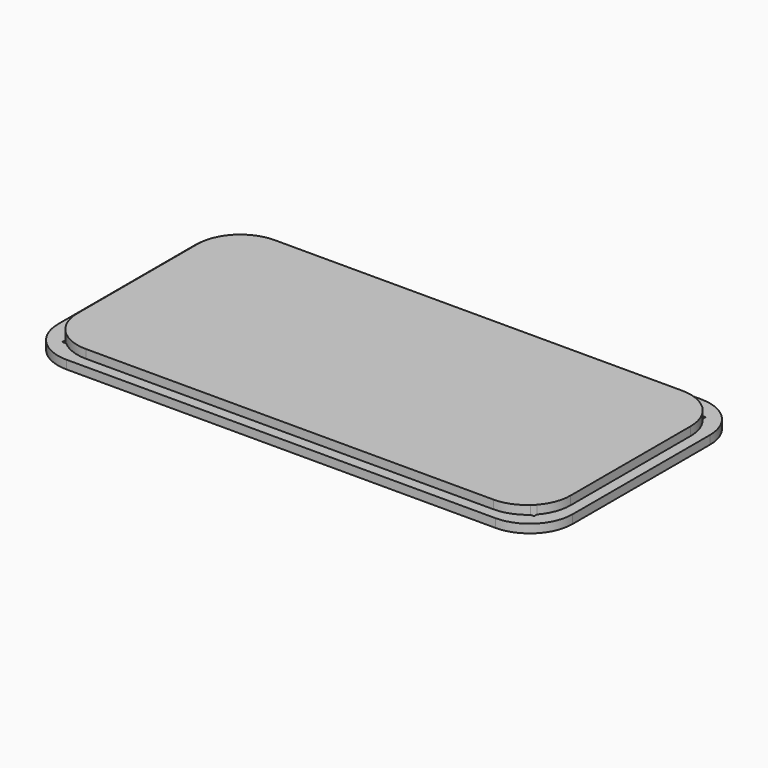
from build123d import *

# Parameters (mm, degrees)
F1_DEPTH = 1
F2_DEPTH = 2


with BuildPart() as f1:
    # F0 (on Top) → F1 (new body)
    with BuildSketch(Plane.XY):
        with BuildLine():
            Line((25, 15), (-25, 15))
            ThreePointArc((-25, 15), (-28.5355339059, 13.5355339059), (-30, 10))
            Line((-30, 10), (-30, -10))
            ThreePointArc((-30, -10), (-28.5355339059, -13.5355339059), (-25, -15))
            Line((-25, -15), (25, -15))
            ThreePointArc((25, -15), (28.5355339059, -13.5355339059), (30, -10))
            Line((30, -10), (30, 10))
            ThreePointArc((30, 10), (28.5355339059, 13.5355339059), (25, 15))
        make_face()
        with BuildLine():
            Line((-27.5, 12.0571891388), (-27.5, 12.5))
            Line((-27.5, 12.5), (-27.0571891388, 12.5))
            ThreePointArc((-27.0571891388, 12.5), (-25.517766953, 13.4270717335), (-23.75, 13.75))
            Line((-23.75, 13.75), (23.75, 13.75))
            ThreePointArc((23.75, 13.75), (25.517766953, 13.4270717335), (27.0571891388, 12.5))
            Line((27.0571891388, 12.5), (27.5, 12.5))
            Line((27.5, 12.5), (27.5, 12.0571891388))
            ThreePointArc((27.5, 12.0571891388), (28.4270717335, 10.517766953), (28.75, 8.75))
            Line((28.75, 8.75), (28.75, -8.75))
            ThreePointArc((28.75, -8.75), (28.4270717335, -10.517766953), (27.5, -12.0571891388))
            Line((27.5, -12.0571891388), (27.5, -12.5))
            Line((27.5, -12.5), (27.0571891388, -12.5))
            ThreePointArc((27.0571891388, -12.5), (25.517766953, -13.4270717335), (23.75, -13.75))
            Line((23.75, -13.75), (-23.75, -13.75))
            ThreePointArc((-23.75, -13.75), (-25.517766953, -13.4270717335), (-27.0571891388, -12.5))
            Line((-27.0571891388, -12.5), (-27.5, -12.5))
            Line((-27.5, -12.5), (-27.5, -12.0571891388))
            ThreePointArc((-27.5, -12.0571891388), (-28.4270717335, -10.517766953), (-28.75, -8.75))
            Line((-28.75, -8.75), (-28.75, 8.75))
            ThreePointArc((-28.75, 8.75), (-28.4270717335, 10.517766953), (-27.5, 12.0571891388))
        make_face(mode=Mode.SUBTRACT)
    extrude(amount=F1_DEPTH)

    # F0 (on Top) → F2 (join)
    with BuildSketch(Plane.XY):
        with BuildLine():
            Line((27.0571891388, 12.5), (-27.0571891388, 12.5))
            ThreePointArc((-27.0571891388, 12.5), (-27.2855339059, 12.2855339059), (-27.5, 12.0571891388))
            Line((-27.5, 12.0571891388), (-27.5, -12.0571891388))
            ThreePointArc((-27.5, -12.0571891388), (-27.2855339059, -12.2855339059), (-27.0571891388, -12.5))
            Line((-27.0571891388, -12.5), (27.0571891388, -12.5))
            ThreePointArc((27.0571891388, -12.5), (27.2855339059, -12.2855339059), (27.5, -12.0571891388))
            Line((27.5, -12.0571891388), (27.5, 12.0571891388))
            ThreePointArc((27.5, 12.0571891388), (27.2855339059, 12.2855339059), (27.0571891388, 12.5))
        make_face()
        with BuildLine():
            ThreePointArc((28.75, 8.75), (28.4270717335, 10.517766953), (27.5, 12.0571891388))
            Line((27.5, 12.0571891388), (27.5, -12.0571891388))
            ThreePointArc((27.5, -12.0571891388), (28.4270717335, -10.517766953), (28.75, -8.75))
            Line((28.75, -8.75), (28.75, 8.75))
        make_face()
        with BuildLine():
            ThreePointArc((-23.75, 13.75), (-25.517766953, 13.4270717335), (-27.0571891388, 12.5))
            Line((-27.0571891388, 12.5), (27.0571891388, 12.5))
            ThreePointArc((27.0571891388, 12.5), (25.517766953, 13.4270717335), (23.75, 13.75))
            Line((23.75, 13.75), (-23.75, 13.75))
        make_face()
        with BuildLine():
            Line((27.0571891388, -12.5), (-27.0571891388, -12.5))
            ThreePointArc((-27.0571891388, -12.5), (-25.517766953, -13.4270717335), (-23.75, -13.75))
            Line((-23.75, -13.75), (23.75, -13.75))
            ThreePointArc((23.75, -13.75), (25.517766953, -13.4270717335), (27.0571891388, -12.5))
        make_face()
        with BuildLine():
            Line((-27.5, -12.0571891388), (-27.5, 12.0571891388))
            ThreePointArc((-27.5, 12.0571891388), (-28.4270717335, 10.517766953), (-28.75, 8.75))
            Line((-28.75, 8.75), (-28.75, -8.75))
            ThreePointArc((-28.75, -8.75), (-28.4270717335, -10.517766953), (-27.5, -12.0571891388))
        make_face()
    extrude(amount=F2_DEPTH)


solid = f1.part
